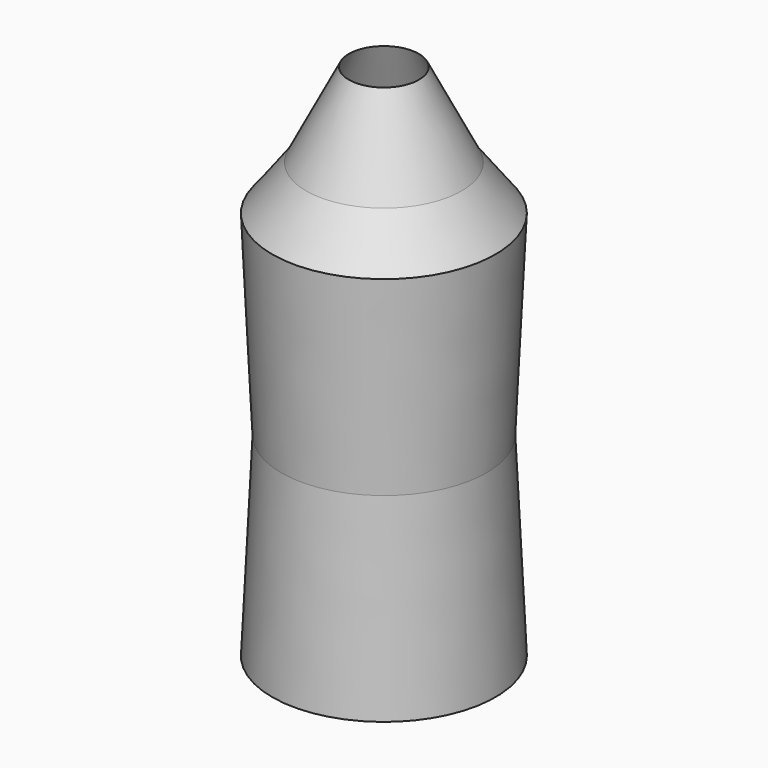
from build123d import *


# Not quite as in the source:
# - a feature names something its author has since deleted; it is built from what else it names


with BuildPart() as f1:
    # F0 (on Front) → F1 (revolve)
    with BuildSketch(Plane.XZ):
        Polygon((-78, 139.9767085075), (-70, 139.9767085075), (-48.5, 189.5767085075), (-64.9242475629, 157.222121954), align=None)
        Polygon((-74.508, -10.1073468104), (-74.508, 14.9767085075), (-70, 14.9767085075), (-70, 64.7767065075), (-70, 139.9767085075), (-78, 139.9767085075), (-74.508, 64.7767065075), (-78, -10.1073468104), align=None)
    revolve(axis=Axis((-35, 0, -12.4232914925), (0, 0, 1)))


solid = f1.part
